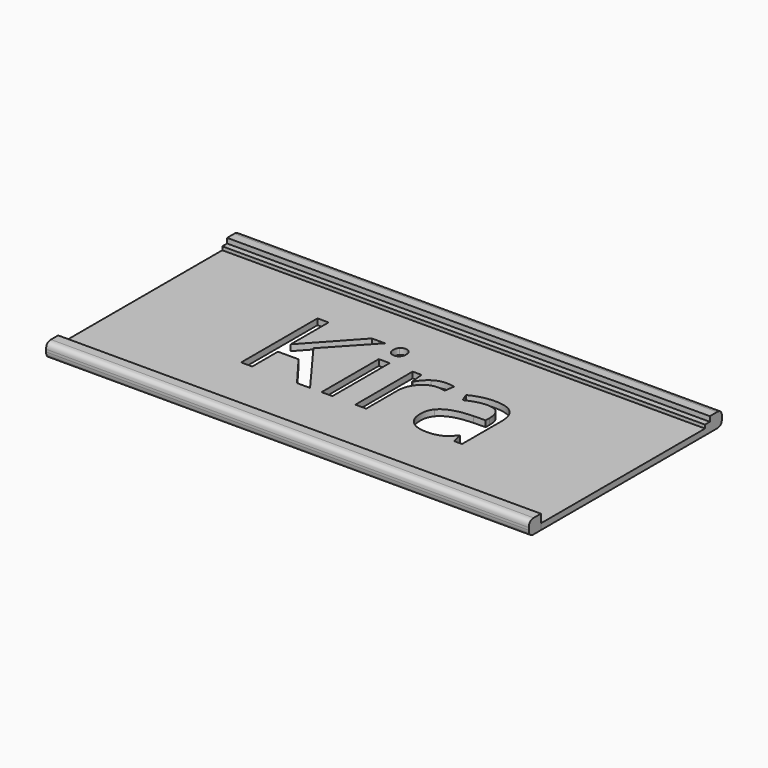
from build123d import *

# Parameters (mm, degrees)
F0_W          = 203.2
F0_H          = 6.35
F1_DEPTH      = 6.096
F0_H_2        = 88.9
F2_DEPTH      = 2.54
F4_DEPTH      = 2.54
F5_T1_DEPTH   = 215.9
F5_2_T1_DEPTH = 215.9


# Not quite as in the source:
# - a fillet or chamfer that OpenCascade refuses, or shapes differently, is made with other operations: its cross-section is extruded or revolved along the edge and cut away or added


with BuildPart() as f1:
    # F0 (on Top) → F1 (new body)
    with BuildSketch(Plane.XY):
        with Locations((-4.4018315911, 50.6631300867)):
            Rectangle(F0_W, F0_H)
    extrude(amount=F1_DEPTH)



with BuildPart() as f1b:
    # F0 (on Top) → F1, piece 2 (new body)
    with BuildSketch(Plane.XY):
        with Locations((-4.4018315911, -44.5868699133)):
            Rectangle(F0_W, F0_H)
    extrude(amount=F1_DEPTH)

    # F5: fillet of radius 2.54 on 2 edges, made by hand

    # F5_s2 → F5_t1 (cut)
    with BuildSketch(Plane.YZ.offset(-112.3518315911)):
        with BuildLine():
            add(Edge.make_bspline(
                [(-47.7618699133, 3.556), (-47.7618699133, 6.096), (-45.2218699133, 6.096)],
                knots=[0, 0, 0, 1, 1, 1], degree=2, weights=[1, 1, 1]))
            Line((-45.2218699133, 6.096), (-47.7618699133, 6.096))
            Line((-47.7618699133, 6.096), (-47.7618699133, 3.556))
        make_face()
        with BuildLine():
            add(Edge.make_bspline(
                [(-47.7618699133, 2.54), (-47.7618699133, 0), (-45.2218699133, 0)],
                knots=[0, 0, 0, 1, 1, 1], degree=2, weights=[1, 1, 1]))
            Line((-45.2218699133, 0), (-47.7618699133, 0))
            Line((-47.7618699133, 0), (-47.7618699133, 2.54))
        make_face()
    extrude(amount=F5_T1_DEPTH, mode=Mode.SUBTRACT)


with BuildPart() as f2:
    # F0 (on Top) → F2 (new body)
    with BuildSketch(Plane.XY):
        with Locations((-4.4018315911, 3.0381300867)):
            Rectangle(F0_W, F0_H_2)
        Polygon((-12.8579193956, 16.5757056756), (-12.8579193956, 0), (-12.8579193956, -13.5469855741), (-17.4224965514, -13.5469855741), (-17.4224965514, 0), (-17.4224965514, 16.5757056756), align=None, mode=Mode.SUBTRACT)
        with BuildLine():
            Line((-3.1834784103, -13.5469855741), (-3.1834784103, 0))
            Line((-3.1834784103, 0), (-3.1834784103, 16.5757056756))
            Line((-3.1834784103, 16.5757056756), (0.5807586276, 16.5757056756))
            Line((0.5807586276, 16.5757056756), (1.1084554086, 10.9997096895))
            Line((1.1084554086, 10.9997096895), (1.3283290674, 10.9997096895))
            add(Edge.make_bspline(
                [(1.3283290674, 10.9997096895), (2.9993688739, 13.9372217705), (5.3652094422, 15.5335045331)],
                knots=[0, 0, 0, 1, 1, 1], degree=2))
            add(Edge.make_bspline(
                [(5.3652094422, 15.5335045331), (7.7310500104, 17.1297872956), (10.5630227352, 17.1297872956)],
                knots=[0, 0, 0, 1, 1, 1], degree=2))
            add(Edge.make_bspline(
                [(10.5630227352, 17.1297872956), (12.568270503, 17.1297872956), (14.1601557924, 16.7955793343)],
                knots=[0, 0, 0, 1, 1, 1], degree=2))
            Line((14.1601557924, 16.7955793343), (13.5269196552, 12.5652101399))
            add(Edge.make_bspline(
                [(13.5269196552, 12.5652101399), (11.6623910289, 12.9785726183), (10.2288147739, 12.9785726183)],
                knots=[0, 0, 0, 1, 1, 1], degree=2))
            add(Edge.make_bspline(
                [(10.2288147739, 12.9785726183), (6.5701170921, 12.9785726183), (3.9756079188, 10.0102782251)],
                knots=[0, 0, 0, 1, 1, 1], degree=2))
            add(Edge.make_bspline(
                [(3.9756079188, 10.0102782251), (1.3810987455, 7.0419838319), (1.3810987455, 2.6181258177)],
                knots=[0, 0, 0, 1, 1, 1], degree=2))
            Line((1.3810987455, 2.6181258177), (1.3810987455, 0))
            Line((1.3810987455, 0), (1.3810987455, -13.5469855741))
            Line((1.3810987455, -13.5469855741), (-3.1834784103, -13.5469855741))
        make_face(mode=Mode.SUBTRACT)
        with BuildLine():
            add(Edge.make_bspline(
                [(17.5462101373, -5.2181713804), (17.5462101373, -2.1025919099), (19.248891356, 0)],
                knots=[0, 0, 0, 0.3416070953, 0.3416070953, 0.3416070953], degree=2))
            add(Edge.make_bspline(
                [(19.248891356, 0), (22.5305364068, 4.0524087886), (32.1370261324, 4.3419353024)],
                knots=[0.3416070953, 0.3416070953, 0.3416070953, 1, 1, 1], degree=2))
            Line((32.1370261324, 4.3419353024), (37.2468899619, 4.509039283))
            Line((37.2468899619, 4.509039283), (37.2468899619, 6.3823628556))
            add(Edge.make_bspline(
                [(37.2468899619, 6.3823628556), (37.2468899619, 9.9267262348), (35.7253642433, 11.615355934)],
                knots=[0, 0, 0, 1, 1, 1], degree=2))
            add(Edge.make_bspline(
                [(35.7253642433, 11.615355934), (34.2038385247, 13.3039856333), (30.8441690189, 13.3039856333)],
                knots=[0, 0, 0, 1, 1, 1], degree=2))
            add(Edge.make_bspline(
                [(30.8441690189, 13.3039856333), (27.079931981, 13.3039856333), (22.3306609518, 10.9997096895)],
                knots=[0, 0, 0, 1, 1, 1], degree=2))
            Line((22.3306609518, 10.9997096895), (20.9234695358, 14.4913033906))
            add(Edge.make_bspline(
                [(20.9234695358, 14.4913033906), (23.1485909624, 15.6962110406), (25.800267287, 16.3822168559)],
                knots=[0, 0, 0, 1, 1, 1], degree=2))
            add(Edge.make_bspline(
                [(25.800267287, 16.3822168559), (28.4519436116, 17.0682226712), (31.1256073021, 17.0682226712)],
                knots=[0, 0, 0, 1, 1, 1], degree=2))
            add(Edge.make_bspline(
                [(31.1256073021, 17.0682226712), (36.5081144684, 17.0682226712), (39.1070211149, 14.6803947371)],
                knots=[0, 0, 0, 1, 1, 1], degree=2))
            add(Edge.make_bspline(
                [(39.1070211149, 14.6803947371), (41.7059277614, 12.292566803), (41.7059277614, 7.0155989928)],
                knots=[0, 0, 0, 1, 1, 1], degree=2))
            Line((41.7059277614, 7.0155989928), (41.7059277614, 0))
            Line((41.7059277614, 0), (41.7059277614, -13.5469855741))
            Line((41.7059277614, -13.5469855741), (38.3198734166, -13.5469855741))
            Line((38.3198734166, -13.5469855741), (37.4139939425, -9.2550517551))
            Line((37.4139939425, -9.2550517551), (37.1941202838, -9.2550517551))
            add(Edge.make_bspline(
                [(37.1941202838, -9.2550517551), (34.9426140181, -12.0870244799), (32.7043001719, -13.094045837)],
                knots=[0, 0, 0, 1, 1, 1], degree=2))
            add(Edge.make_bspline(
                [(32.7043001719, -13.094045837), (30.4659863258, -14.1010671941), (27.10631682, -14.1010671941)],
                knots=[0, 0, 0, 1, 1, 1], degree=2))
            add(Edge.make_bspline(
                [(27.10631682, -14.1010671941), (22.6296891277, -14.1010671941), (20.0879496325, -11.787996304)],
                knots=[0, 0, 0, 1, 1, 1], degree=2))
            add(Edge.make_bspline(
                [(20.0879496325, -11.787996304), (17.5462101373, -9.4749254139), (17.5462101373, -5.2181713804)],
                knots=[0, 0, 0, 1, 1, 1], degree=2))
        make_face(mode=Mode.SUBTRACT)
        Polygon((-39.0228847876, 9.179155795), (-32.2521916973, 0), (-22.259717044, -13.5469855741), (-27.7565585129, -13.5469855741), (-37.9351374754, 0), (-46.6129234879, 0), (-46.6129234879, -13.5469855741), (-51.2830399999, -13.5469855741), (-51.2830399999, 0), (-51.2830399999, 26.6371243003), (-46.6129234879, 26.6371243003), (-46.6129234879, 6.7077758706), (-28.3897946501, 26.6371243003), (-22.8665683422, 26.6371243003), align=None, mode=Mode.SUBTRACT)
        with BuildLine():
            add(Edge.make_bspline(
                [(-17.0399163851, 22.4419348912), (-17.8094741908, 23.1983002773), (-17.8094741908, 24.7374158886)],
                knots=[0, 0, 0, 1, 1, 1], degree=2))
            add(Edge.make_bspline(
                [(-17.8094741908, 24.7374158886), (-17.8094741908, 26.302916339), (-17.0399163851, 27.032896886)],
                knots=[0, 0, 0, 1, 1, 1], degree=2))
            add(Edge.make_bspline(
                [(-17.0399163851, 27.032896886), (-16.2703585795, 27.7628774331), (-15.1094256612, 27.7628774331)],
                knots=[0, 0, 0, 1, 1, 1], degree=2))
            add(Edge.make_bspline(
                [(-15.1094256612, 27.7628774331), (-14.0100573675, 27.7628774331), (-13.2141147228, 27.0197044665)],
                knots=[0, 0, 0, 1, 1, 1], degree=2))
            add(Edge.make_bspline(
                [(-13.2141147228, 27.0197044665), (-12.4181720781, 26.2765314999), (-12.4181720781, 24.7374158886)],
                knots=[0, 0, 0, 1, 1, 1], degree=2))
            add(Edge.make_bspline(
                [(-12.4181720781, 24.7374158886), (-12.4181720781, 23.1983002773), (-13.2141147228, 22.4419348912)],
                knots=[0, 0, 0, 1, 1, 1], degree=2))
            add(Edge.make_bspline(
                [(-13.2141147228, 22.4419348912), (-14.0100573675, 21.6855695051), (-15.1094256612, 21.6855695051)],
                knots=[0, 0, 0, 1, 1, 1], degree=2))
            add(Edge.make_bspline(
                [(-15.1094256612, 21.6855695051), (-16.2703585795, 21.6855695051), (-17.0399163851, 22.4419348912)],
                knots=[0, 0, 0, 1, 1, 1], degree=2))
        make_face(mode=Mode.SUBTRACT)
    extrude(amount=F2_DEPTH)


with BuildPart() as f1_1:
    add(f1.part)

    add(f2.part)  # F4 merges F2
    # F3 (on face) → F4 (join)
    with BuildSketch(Plane.XZ.offset(-47.4881300867)):
        Polygon((97.1981684089, 4.0059988387), (-106.0018315911, 4.0059988387), (-106.0018315911, 2.044348279), (-48.8064140081, 2.044348279), (97.1981684089, 2.044348279), align=None)
    extrude(amount=F4_DEPTH)

    # F5#2: fillet of radius 2.54 on 2 edges, made by hand

    # F5_2_s2 → F5_2_t1 (cut)
    with BuildSketch(Plane.YZ.offset(-112.3518315911)):
        with BuildLine():
            add(Edge.make_bspline(
                [(51.2981300867, 6.096), (53.8381300867, 6.096), (53.8381300867, 3.556)],
                knots=[0, 0, 0, 1, 1, 1], degree=2, weights=[1, 1, 1]))
            Line((53.8381300867, 3.556), (53.8381300867, 6.096))
            Line((53.8381300867, 6.096), (51.2981300867, 6.096))
        make_face()
        with BuildLine():
            add(Edge.make_bspline(
                [(53.8381300867, 2.54), (53.8381300867, 0), (51.2981300867, 0)],
                knots=[0, 0, 0, 1, 1, 1], degree=2, weights=[1, 1, 1]))
            Line((51.2981300867, 0), (53.8381300867, 0))
            Line((53.8381300867, 0), (53.8381300867, 2.54))
        make_face()
    extrude(amount=F5_2_T1_DEPTH, mode=Mode.SUBTRACT)


solid = Compound([f1b.part, f1_1.part])
